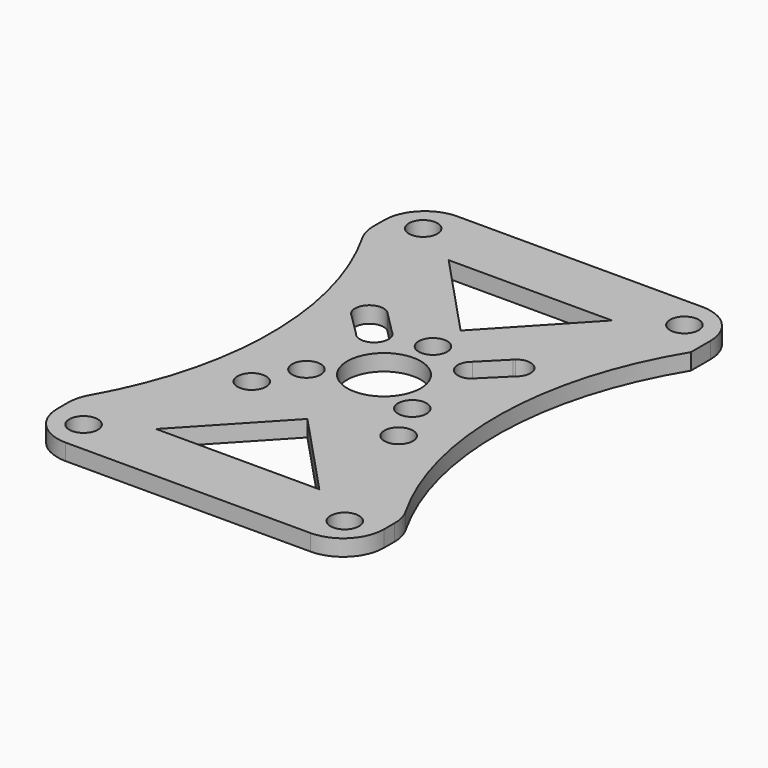
from build123d import *

# Parameters (mm, degrees)
F0_R     = 1.75
F0_R_2   = 4.5
F1_DEPTH = 2
F2_R     = 5


with BuildPart() as f1:
    # F0 (on Top) → F1 (new body)
    with BuildSketch(Plane.XY):
        with BuildLine():
            Line((20, 30), (-20, 30))
            Line((-20, 30), (-20, 22))
            ThreePointArc((-20, 22), (-13.8300253787, 0), (-20, -22))
            Line((-20, -22), (-20, -30))
            Line((-20, -30), (20, -30))
            Line((20, -30), (20, -22))
            ThreePointArc((20, -22), (13.8300253787, 0), (20, 22))
            Line((20, 22), (20, 30))
        make_face()
        with Locations((-16, -26)):
            Circle(F0_R, mode=Mode.SUBTRACT)
        with Locations((-9, -9)):
            Circle(F0_R, mode=Mode.SUBTRACT)
        with Locations((-6.4855394704, -3.7666666667)):
            Circle(F0_R, mode=Mode.SUBTRACT)
        Polygon((10, -22.4003139883), (0, -22.4003139883), (-10, -22.4003139883), (0, -11.7255505174), align=None, mode=Mode.SUBTRACT)
        with Locations((16, -26)):
            Circle(F0_R, mode=Mode.SUBTRACT)
        with Locations((9, -9)):
            Circle(F0_R, mode=Mode.SUBTRACT)
        with Locations((6.4855394704, -3.7666666667)):
            Circle(F0_R, mode=Mode.SUBTRACT)
        with BuildLine():
            ThreePointArc((-10.4007968114, 7.9510632559), (-10.1861204729, 10.2867082901), (-7.840755933, 10.310974139))
            ThreePointArc((-7.840755933, 10.310974139), (-7.7595664935, 10.2344329532), (-7.6834199086, 10.1528733074))
            Line((-7.6834199086, 10.1528733074), (-4.9243436791, 7.3803852648))
            ThreePointArc((-4.9243436791, 7.3803852648), (-4.4275976085, 6.7681475895), (-4.25, 6))
            ThreePointArc((-4.25, 6), (-5.1630952479, 4.4630906221), (-6.9495319267, 4.5300037006))
            ThreePointArc((-6.9495319267, 4.5300037006), (-7.2319861689, 4.7571363391), (-7.4615928772, 5.0375831146))
            Line((-7.4615928772, 5.0375831146), (-10.0365828557, 7.5900368858))
            ThreePointArc((-10.0365828557, 7.5900368858), (-10.2319861689, 7.7571363391), (-10.4007968114, 7.9510632559))
        make_face(mode=Mode.SUBTRACT)
        with Locations((-16, 26)):
            Circle(F0_R, mode=Mode.SUBTRACT)
        Circle(F0_R_2, mode=Mode.SUBTRACT)
        with Locations((0, 7.5)):
            Circle(F0_R, mode=Mode.SUBTRACT)
        with BuildLine():
            ThreePointArc((7.840755933, 10.310974139), (9.7189655356, 10.5954900685), (10.75, 9))
            ThreePointArc((10.75, 9), (10.6604057365, 8.4472317031), (10.4007968114, 7.9510632559))
            ThreePointArc((10.4007968114, 7.9510632559), (10.2319861689, 7.7571363391), (10.0365828557, 7.5900368858))
            Line((10.0365828557, 7.5900368858), (7.4615928772, 5.0375831146))
            ThreePointArc((7.4615928772, 5.0375831146), (7.2319861689, 4.7571363391), (6.9495319267, 4.5300037006))
            ThreePointArc((6.9495319267, 4.5300037006), (4.5734147043, 4.9864150781), (4.9243436791, 7.3803852648))
            Line((4.9243436791, 7.3803852648), (7.6834199086, 10.1528733074))
            ThreePointArc((7.6834199086, 10.1528733074), (7.7595664935, 10.2344329532), (7.840755933, 10.310974139))
        make_face(mode=Mode.SUBTRACT)
        Polygon((0, 22.4003139883), (10, 22.4003139883), (0, 11.7255505174), (-10, 22.4003139883), align=None, mode=Mode.SUBTRACT)
        with Locations((16, 26)):
            Circle(F0_R, mode=Mode.SUBTRACT)
    extrude(amount=F1_DEPTH)

    # F2
    f2_edges = [f1.edges().sort_by_distance(p)[0] for p in [
        (-20, 30, 1),
        (-20, -30, 1),
        (20, -30, 1),
        (20, 30, 1),
        (20, -22, 1),
        (-20, -22, 1),
        (-20, 22, 1),
    ]]
    fillet(f2_edges, radius=F2_R)


solid = f1.part
